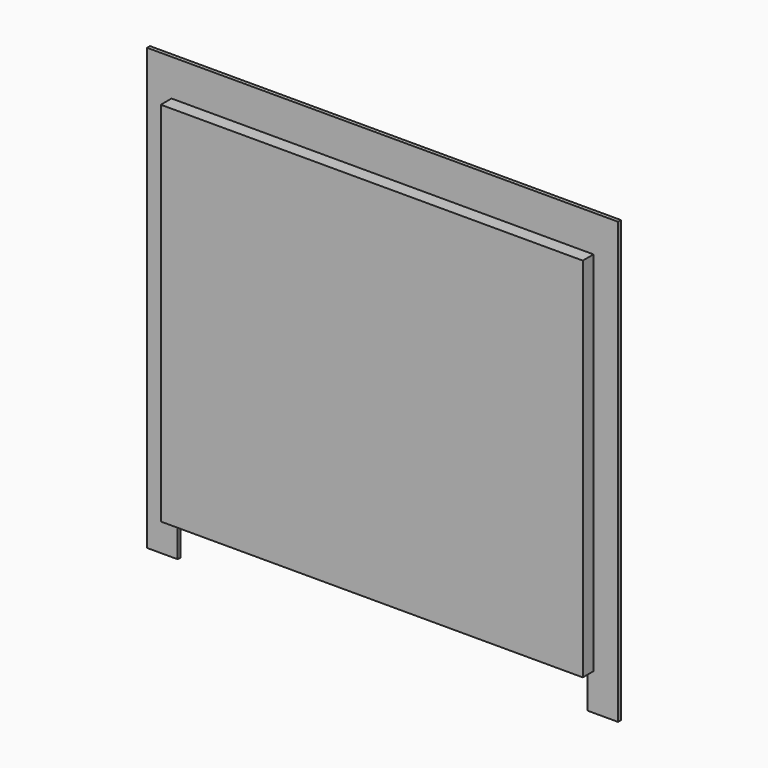
from build123d import *

# Parameters (mm, degrees)
F0_W        = 192.5
F0_H        = 180
F1_DEPTH    = 1.5
F2_W        = 172.5
F2_H        = 150
F3_DEPTH    = 5.5
F4_T        = 2.5
F4_T3_DEPTH = 155
F4_T5_DEPTH = 177.5
F6_W        = 167.5
F6_H        = 4.5
F7_DEPTH    = 17.501


# Not quite as in the source:
# - a shell that OpenCascade refuses in one call is made with other operations: the cavity is built on its own and cut out


with BuildPart() as f1:
    # F0 (on Front) → F1 (new body)
    with BuildSketch(Plane.XZ):
        Rectangle(F0_W, F0_H)
    extrude(amount=F1_DEPTH)

    # F2 (on face) → F3 (join)
    with BuildSketch(Plane.XZ.offset(1.5)):
        Rectangle(F2_W, F2_H)
    extrude(amount=F3_DEPTH)

    # F4: shell of thickness 2.5, made by hand


with BuildPart() as f4_core1:
    # F4_t2: copy of F1
    add(f1.part)

    # the walls: a layer under each face that stays
    f4_faces = [f4_core1.faces().sort_by_distance(p)[0] for p in [
        (96.25, -0.75, 0),
        (0, -0.75, -90),
        (0, -0.75, 90),
        (-82.5, -1.5, -77.1428571429),
        (-96.25, -0.75, 0),
        (86.25, -4.25, 0),
        (0, -4.25, 75),
        (-86.25, -4.25, 0),
        (0, -4.25, -75),
        (0, -7, 0),
    ]]
    thicken(f4_faces, amount=-F4_T, mode=Mode.SUBTRACT)

    # F4_s4 → F4_t3 (cut)
    with BuildSketch(Plane.XY.offset(-77.5)):
        Polygon((86.275, -1.525), (86.25, 1), (83.75, 1), (83.75, -1.5), align=None)
        Polygon((-86.275, -1.525), (-86.25, 1), (-83.75, 1), (-83.75, -1.5), align=None)
    extrude(amount=F4_T3_DEPTH, mode=Mode.SUBTRACT)

    # F4_s6 → F4_t5 (cut)
    with BuildSketch(Plane.YZ.offset(-88.75)):
        Polygon((-1.525, 75.025), (1, 75), (1, 72.5), (-1.5, 72.5), align=None)
        Polygon((-1.525, -75.025), (1, -75), (1, -72.5), (-1.5, -72.5), align=None)
    extrude(amount=F4_T5_DEPTH, mode=Mode.SUBTRACT)


with BuildPart() as f1_1:
    add(f1.part)

    # what is left inside the walls is the cavity
    f4_cavity = [f4_core1.part.solids().sort_by_distance(p)[0] for p in [
        (0, -0.025, -24.166667),
    ]]
    add(f4_cavity, mode=Mode.SUBTRACT)

    # F6 (on face) → F7 (cut, through all)
    with BuildSketch(Plane(origin=(0, 0, -72.5), x_dir=(1, 0, 0), z_dir=(0, 0, -1))):
        with Locations((0, 2.25)):
            Rectangle(F6_W, F6_H)
    extrude(amount=F7_DEPTH, mode=Mode.SUBTRACT)


solid = f1_1.part
